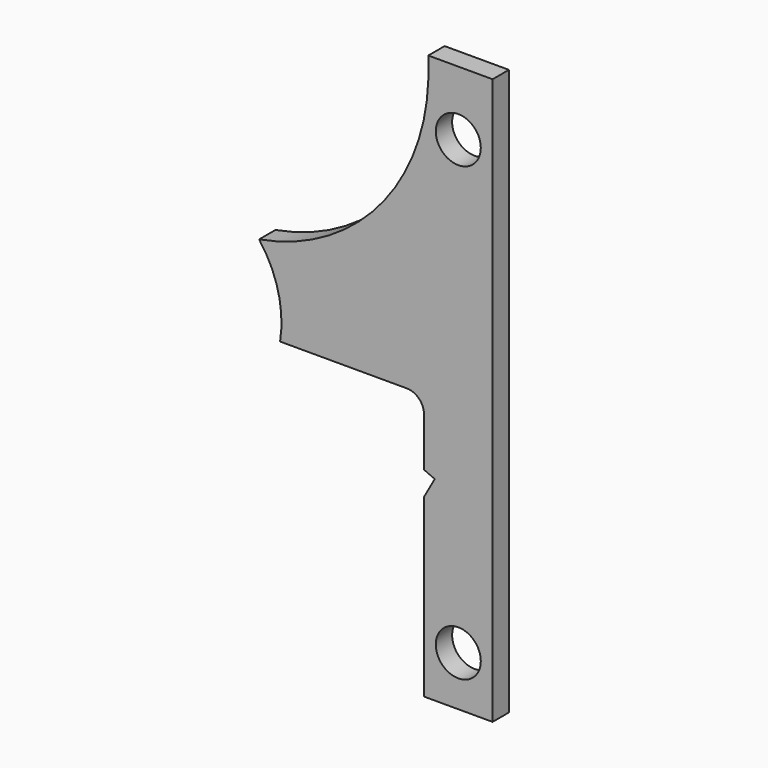
from build123d import *

# Parameters (mm, degrees)
F0_R     = 5.2500022
F1_DEPTH = 4.7625


# Not quite as in the source:
# - ends of sketch curves that miss each other by under 0.0002 mm in the source are joined


with BuildPart() as f1:
    # F0 (on Front) → F1 (new body)
    with BuildSketch(Plane.XZ):
        with BuildLine():
            Line((12.2383296, 65.999995), (12.2383296, 60.9999796))
            ThreePointArc((12.2383296, 60.9999796), (0.5785907755, 31.2052232969), (-27.2383496091, 15.3971707597))
            ThreePointArc((-27.2383496091, 15.3971707597), (-22.7846228753, 6.2046372562), (-22.3335718073, -4.0000195199))
            Line((-22.3335718073, -4.0000195199), (7.2383142, -4.0000174))
            ThreePointArc((7.2383142, -4.0000174), (10.0667356679, -5.1715879321), (11.2383062, -8.0000094))
            Line((11.2383062, -8.0000094), (11.2383316, -19.3998596))
            Line((11.2383316, -19.3998596), (13.7383266, -20.5000098))
            Line((13.7383266, -20.5000098), (11.2383316, -24.9706384))
            Line((11.2383316, -24.9706384), (11.2383316, -65.999995))
            Line((11.2383316, -65.999995), (27.238325, -65.999995))
            Line((27.238325, -65.999995), (27.238325, 65.999995))
            Line((27.238325, 65.999995), (12.2383296, 65.999995))
        make_face()
        with Locations((19.2383156, -54.4085272)):
            Circle(F0_R, mode=Mode.SUBTRACT)
        with Locations((19.2383156, 50.9999996)):
            Circle(F0_R, mode=Mode.SUBTRACT)
    extrude(amount=F1_DEPTH)


solid = f1.part
